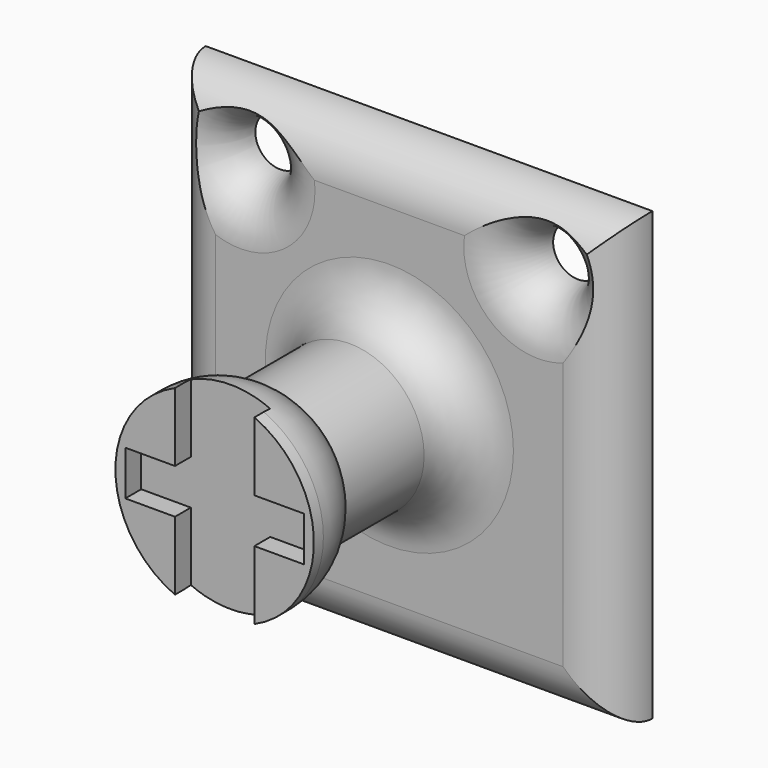
from build123d import *

# Parameters (mm, degrees)
F0_R        = 7.5
F1_DEPTH    = 20
F0_W        = 45
F0_H        = 45
F2_DEPTH    = 5
F3_R        = 2.5
F4_DEPTH    = 25
F5_R        = 10
F5_R_2      = 7.5
F6_DEPTH    = 7
F7_W        = 8
F7_H        = 9.7702028193
F7_W_2      = 5
F7_H_2      = 4.5
F8_DEPTH    = 2
F9_T3_DEPTH = 70
F9_T5_DEPTH = 70


# Not quite as in the source:
# - a fillet or chamfer that OpenCascade refuses, or shapes differently, is made with other operations: its cross-section is extruded or revolved along the edge and cut away or added


with BuildPart() as f1:
    # F0 (on Front) → F1 (new body)
    with BuildSketch(Plane.XZ):
        with Locations((-2.8196598027, -8.5107027553)):
            Circle(F0_R)
    extrude(amount=F1_DEPTH)

    # F0 (on Front) → F2 (join)
    with BuildSketch(Plane.XZ):
        with Locations((-2.8196598027, -8.5107027553)):
            Rectangle(F0_W, F0_H)
        with Locations((-2.8196598027, -8.5107027553)):
            Circle(F0_R, mode=Mode.SUBTRACT)
    extrude(amount=F2_DEPTH)

    # F3 (on face) → F4 (cut)
    with BuildSketch(Plane.XZ.offset(5)):
        with Locations((12.1803401973, 7.9892972447)):
            Circle(F3_R)
        with Locations((-17.8196598027, 7.9892972447)):
            Circle(F3_R)
    extrude(amount=-F4_DEPTH, mode=Mode.SUBTRACT)

    # F5 (on face) → F6 (join)
    with BuildSketch(Plane.XZ.offset(20)):
        with Locations((-2.8196598027, -8.5107027553)):
            Circle(F5_R)
        with Locations((-2.8196598027, -8.5107027553)):
            Circle(F5_R_2, mode=Mode.SUBTRACT)
        with Locations((-2.8196598027, -8.5107027553)):
            Circle(F5_R_2)
    extrude(amount=F6_DEPTH)

    # F7 (on face) → F8 (cut)
    with BuildSketch(Plane.XZ.offset(27)):
        with Locations((-2.8196598027, -15.6458041649)):
            Rectangle(F7_W, F7_H)
        with Locations((-9.3196598027, -8.5107027553)):
            Rectangle(F7_W_2, F7_H_2)
        with Locations((-2.8196598027, -8.5107027553)):
            Rectangle(F7_W, F7_H_2)
        with Locations((3.6803401973, -8.5107027553)):
            Rectangle(F7_W_2, F7_H_2)
        with Locations((-2.8196598027, -1.3756013457)):
            Rectangle(F7_W, F7_H)
    extrude(amount=-F8_DEPTH, mode=Mode.SUBTRACT)

    # F9: fillet of radius 5 on 7 edges, made by hand

    # F9_s1 → F9_t2 (revolve)
    with BuildSketch(Plane.XY.offset(-8.5107027553)):
        with BuildLine():
            ThreePointArc((4.6803401973, -10), (6.1448062914, -6.4644660941), (9.6803401973, -5))
            Line((9.6803401973, -5), (4.6803401973, -5))
            Line((4.6803401973, -5), (4.6803401973, -10))
        make_face()
    revolve(axis=Axis((-2.8196598027, -5, -8.5107027553), (0, -1, 0)))

    # F9_s4 → F9_t3 (cut)
    with BuildSketch(Plane.YZ.offset(-37.8196598027)):
        with BuildLine():
            ThreePointArc((-5, 8.9892972447), (-3.5355339059, 12.5248311506), (0, 13.9892972447))
            Line((0, 13.9892972447), (-5, 13.9892972447))
            Line((-5, 13.9892972447), (-5, 8.9892972447))
        make_face()
        with BuildLine():
            ThreePointArc((-5, -26.0107027553), (-3.5355339059, -29.5462366612), (0, -31.0107027553))
            Line((0, -31.0107027553), (-5, -31.0107027553))
            Line((-5, -31.0107027553), (-5, -26.0107027553))
        make_face()
    extrude(amount=F9_T3_DEPTH, mode=Mode.SUBTRACT)

    # F9_s6 → F9_t5 (cut)
    with BuildSketch(Plane.XY.offset(-43.5107027553)):
        with BuildLine():
            ThreePointArc((14.6803401973, -5), (18.2158741033, -3.5355339059), (19.6803401973, 0))
            Line((19.6803401973, 0), (19.6803401973, -5))
            Line((19.6803401973, -5), (14.6803401973, -5))
        make_face()
        with BuildLine():
            ThreePointArc((-20.3196598027, -5), (-23.8551937086, -3.5355339059), (-25.3196598027, 0))
            Line((-25.3196598027, 0), (-25.3196598027, -5))
            Line((-25.3196598027, -5), (-20.3196598027, -5))
        make_face()
    extrude(amount=F9_T5_DEPTH, mode=Mode.SUBTRACT)

    # F9_s7 → F9_t8 (revolve, cut)
    with BuildSketch(Plane.XY.offset(7.9892972447)):
        with BuildLine():
            ThreePointArc((-10.3196598027, -5), (-13.8551937086, -3.5355339059), (-15.3196598027, 0))
            Line((-15.3196598027, 0), (-15.3196598027, -5))
            Line((-15.3196598027, -5), (-10.3196598027, -5))
        make_face()
    revolve(axis=Axis((-17.8196598027, -5, 7.9892972447), (0, -1, 0)), mode=Mode.SUBTRACT)

    # F9_s9 → F9_t10 (revolve, cut)
    with BuildSketch(Plane.XY.offset(7.9892972447)):
        with BuildLine():
            ThreePointArc((19.6803401973, -5), (16.1448062914, -3.5355339059), (14.6803401973, 0))
            Line((14.6803401973, 0), (14.6803401973, -5))
            Line((14.6803401973, -5), (19.6803401973, -5))
        make_face()
    revolve(axis=Axis((12.1803401973, -5, 7.9892972447), (0, -1, 0)), mode=Mode.SUBTRACT)

    # F10: fillet of radius 8 on 1 edges, made by hand

    # F10_s1 → F10_t2 (revolve, cut)
    with BuildSketch(Plane.XY.offset(-8.5107027553)):
        with BuildLine():
            ThreePointArc((7.1803401973, -25.8094750193), (6.5288094257, -22.6471973591), (4.6803401973, -20))
            Line((4.6803401973, -20), (7.1803401973, -20))
            Line((7.1803401973, -20), (7.1803401973, -25.8094750193))
        make_face()
    revolve(axis=Axis((-2.8196598027, -20, -8.5107027553), (0, -1, 0)), mode=Mode.SUBTRACT)


solid = f1.part
